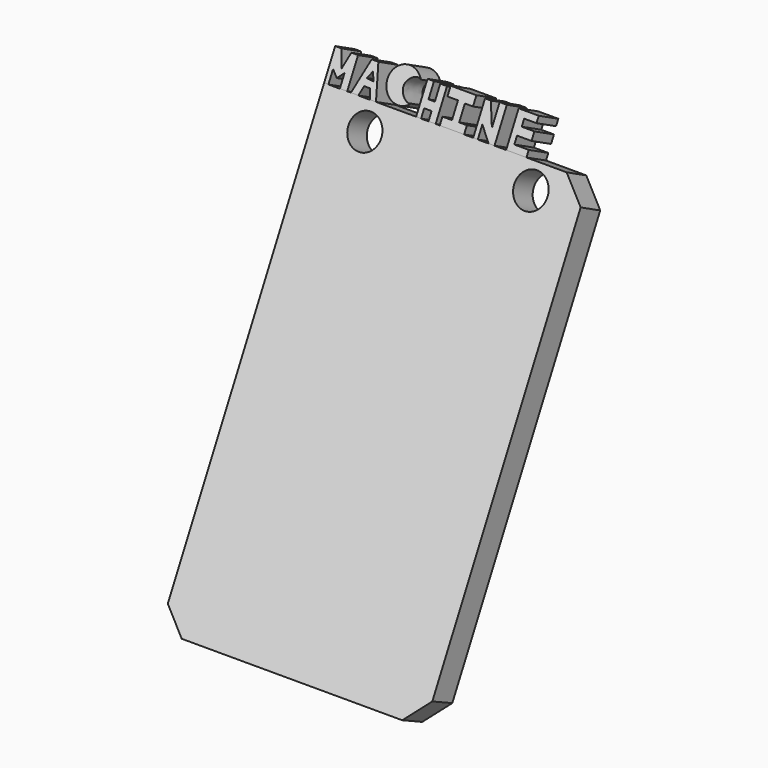
from build123d import *

# Parameters (mm, degrees)
F1_DEPTH = 60.96
F2_R     = 3.81
F2_R_2   = 3.8508677483
F3_DEPTH = 25.4
F5_DEPTH = 6.35
F7_DEPTH = 25.4
F8_SIZE  = 5.08


with BuildPart() as f1:
    # F0 (on Right) → F1 (new body)
    with BuildSketch(Plane.YZ):
        Polygon((-48.4152159798, -43.2849022093), (-1.161592304, 48.3728786074), (-6.805678506, 51.2826536751), (-54.1754523457, -40.600423435), align=None)
    extrude(amount=F1_DEPTH)

    # F2 (on face) → F3 (cut)
    with BuildSketch(Plane(origin=(0, -26.263645076, 13.5400659902), x_dir=(1, 0, 0), z_dir=(0, -0.8888324728, 0.4582322941))):
        with Locations((11.4869037643, 36.7000326514)):
            Circle(F2_R)
        with Locations((49.5869037643, 37.1220372617)):
            Circle(F2_R_2)
    extrude(amount=-F3_DEPTH, mode=Mode.SUBTRACT)

    # F4 (on face) → F5 (join)
    with BuildSketch(Plane(origin=(0, -20.619558874, 10.6302909225), x_dir=(-1, 0, 0), z_dir=(0, 0.8888324728, -0.4582322941))):
        Polygon((-5.3176167421, 42.4631062004), (0, 42.4631062004), (0, 49.383803788), (-1.4188548084, 49.383803788), (-2.7015644591, 45.8769905897), (-3.7731891498, 49.2842938335), (-5.3176167421, 49.2842938335), align=None)
        Polygon((-11.942232959, 42.4631062004), (-6.1762407422, 42.4631062004), (-8.4014460444, 49.4251023562), (-9.9458741024, 49.4251023562), align=None)
        Polygon((-25.6943982095, 42.4631062004), (-21.1968142539, 42.4631062004), (-21.1968142539, 49.6102381082), (-22.6909797639, 49.6102381082), (-22.6909797639, 46.1899932058), (-24.135671556, 46.1899932058), (-24.135671556, 49.5950202973), (-25.6943982095, 49.5950202973), align=None)
        Polygon((-46.6139614582, 43.8990030022), (-46.6139614582, 42.4631062004), (-41.936211288, 42.4631062004), (-41.936211288, 50.3241378398), (-46.5652421117, 50.3241378398), (-46.5652421117, 48.9213052721), (-43.7149144709, 48.9213052721), (-43.7149144709, 47.3909783693), (-46.6309636831, 47.3909783693), (-46.6309636831, 45.5906685026), (-43.2935357094, 45.5906685026), (-43.2935357094, 43.8990030022), align=None)
        Polygon((-32.2451777756, 42.4631062004), (-26.6419369727, 42.4631062004), (-26.6419369727, 44.1295947464), (-28.852455318, 44.1295947464), (-28.852455318, 47.8782388897), (-26.4258272946, 47.8782388897), (-26.4258272946, 49.8971711429), (-29.0248729289, 49.8971711429), (-32.3545746505, 49.8971711429), (-32.3545746505, 47.7699819537), (-30.4757487029, 47.7699819537), (-30.4757487029, 44.2036125393), (-32.2451777756, 44.2036125393), align=None)
        Polygon((-39.2559804022, 50.1821931036), (-39.2559804022, 42.4631062004), (-34.3486145139, 42.4631062004), (-34.3486145139, 49.8971711429), (-35.6831140816, 49.8971711429), (-37.6087278128, 45.307162735), (-37.6087278128, 50.1821931036), align=None)
    extrude(amount=-F5_DEPTH)

    # F6 (on face) → F7 (cut)
    with BuildSketch(Plane(origin=(0, -26.263645076, 13.5400659902), x_dir=(1, 0, 0), z_dir=(0, -0.8888324728, 0.4582322941))):
        Polygon((0.9895682648, 45.3476009629), (0.9914431559, 42.433750795), (3.6224654218, 42.435443703), (3.6224654218, 45.3893982965), (2.3443866521, 44.0524443984), align=None)
        Polygon((35.3990507247, 45.3338064253), (35.3990507247, 42.4558900654), (37.8731534896, 42.457482005), align=None)
        Polygon((22.3342671491, 44.4084667024), (22.3355289257, 42.447484458), (24.0494933407, 42.4485872932), (24.048231564, 44.4095695376), align=None)
        Polygon((8.5106072947, 44.4005616009), (7.8737791451, 42.4381791732), (10.5184626663, 42.4398808714), (9.8749566823, 44.4005616009), align=None)
        Polygon((10.1390406489, 45.7629784942), (9.4444689872, 47.4718217689), (8.5177887231, 45.9441042783), align=None)
    extrude(amount=-F7_DEPTH, mode=Mode.SUBTRACT)

    # F8
    f8_edges = [f1.edges().sort_by_distance(p)[0] for p in [
        (60.96, -3.983635, 49.827766),
        (60.96, -51.295334, -41.942663),
        (0, -51.295334, -41.942663),
    ]]
    chamfer(f8_edges, length=F8_SIZE)


with BuildPart() as f5:
    # F4 (on face) → F5, piece 2 (new body)
    with BuildSketch(Plane(origin=(0, -20.619558874, 10.6302909225), x_dir=(-1, 0, 0), z_dir=(0, 0.8888324728, -0.4582322941))):
        with BuildLine():
            add(Edge.make_bspline(
                [(-19.8659427695, 49.0752757694), (-18.9275712513, 49.8099196351), (-14.7540508214, 47.2898812626), (-18.2328673452, 43.8742258683), (-19.3155179804, 44.3723326013)],
                knots=[0, 0, 0, 0, 0.3205550369, 0.6411100737, 0.6411100737, 0.6411100737, 0.6411100737], degree=3))
            ThreePointArc((-19.3155179804, 44.3723326013), (-12.9152251226, 47.5050944198), (-19.8659427695, 49.0752757694))
        make_face()
    extrude(amount=-F5_DEPTH)


solid = Compound([f1.part, f5.part])
